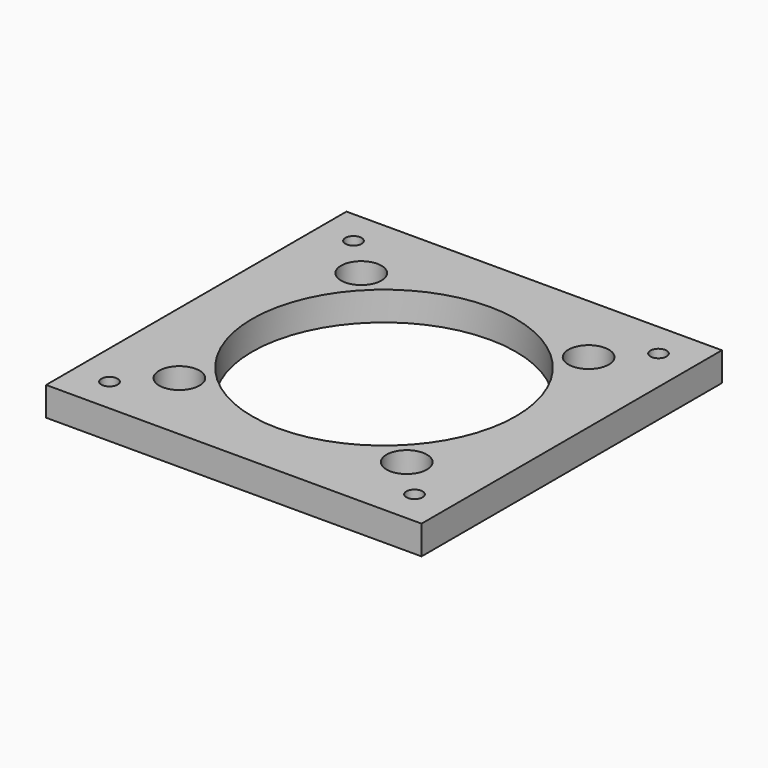
from build123d import *

# Parameters (mm, degrees)
F0_W     = 82.55
F0_H     = 82.55
F0_R     = 1.778
F0_R_2   = 4.445
F0_R_3   = 28.9941
F1_DEPTH = 6.35


# Not quite as in the source:
# - a length typed as a fraction of an inch, garbled in the dataset ("3 / 203.2 mm" for 3/8 in), is restored


with BuildPart() as f1:
    # F0 (on Top) → F1 (new body)
    with BuildSketch(Plane.XY):
        Rectangle(F0_W, F0_H)
        with Locations((-33.528, -33.528)):
            Circle(F0_R, mode=Mode.SUBTRACT)
        with Locations((-24.9936, -24.9936)):
            Circle(F0_R_2, mode=Mode.SUBTRACT)
        with Locations((33.528, -33.528)):
            Circle(F0_R, mode=Mode.SUBTRACT)
        with Locations((24.9936, -24.9936)):
            Circle(F0_R_2, mode=Mode.SUBTRACT)
        with Locations((-24.9936, 24.9936)):
            Circle(F0_R_2, mode=Mode.SUBTRACT)
        with Locations((-33.528, 33.528)):
            Circle(F0_R, mode=Mode.SUBTRACT)
        Circle(F0_R_3, mode=Mode.SUBTRACT)
        with Locations((24.9936, 24.9936)):
            Circle(F0_R_2, mode=Mode.SUBTRACT)
        with Locations((33.528, 33.528)):
            Circle(F0_R, mode=Mode.SUBTRACT)
    extrude(amount=F1_DEPTH)


solid = f1.part
